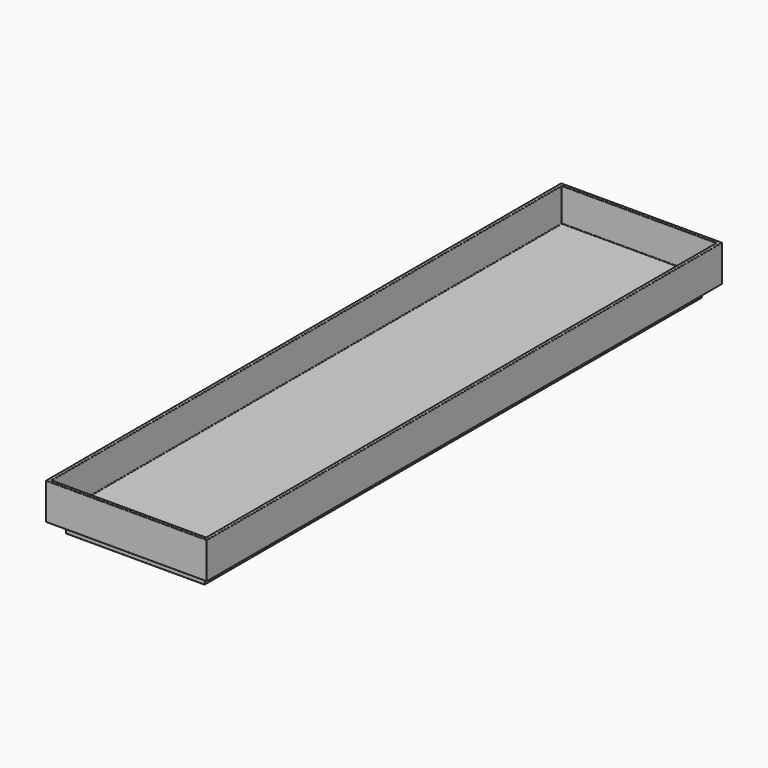
from build123d import *

# Parameters (mm, degrees)
F0_W     = 145
F0_H     = 580
F1_DEPTH = 3
F2_W     = 145
F2_H     = 580
F2_W_2   = 138.9999985695
F2_H_2   = 573.9999985695
F3_DEPTH = 30
F4_W     = 125
F4_H     = 560
F4_W_2   = 119.0000200272
F4_H_2   = 554.0000200272
F5_DEPTH = 10
F6_R     = 0.5


with BuildPart() as f1:
    # F0 (on Top) → F1 (new body)
    with BuildSketch(Plane.XY):
        Rectangle(F0_W, F0_H)
    extrude(amount=F1_DEPTH)

    # F2 (on face) → F3 (join)
    with BuildSketch(Plane.XY.offset(3)):
        Rectangle(F2_W, F2_H)
        Rectangle(F2_W_2, F2_H_2, mode=Mode.SUBTRACT)
    extrude(amount=F3_DEPTH)

    # F4 (on face) → F5 (join)
    with BuildSketch(Plane(origin=(0, 0, 0), x_dir=(1, 0, 0), z_dir=(0, 0, -1))):
        Rectangle(F4_W, F4_H)
        Rectangle(F4_W_2, F4_H_2, mode=Mode.SUBTRACT)
    extrude(amount=F5_DEPTH)

    # F6
    f6_edges = [f1.edges().sort_by_distance(p)[0] for p in [
        (0, 290, 0),
        (72.5, 0, 0),
        (-72.5, 0, 0),
        (0, -290, 0),
        (62.5, 0, 0),
        (0, 280, 0),
        (-62.5, 0, 0),
        (0, -280, 0),
        (59.50001, 0, 0),
        (0, -277.00001, 0),
        (-59.50001, 0, 0),
        (0, 277.00001, 0),
        (-62.5, 280, -5),
        (0, -280, -10),
        (-62.5, 0, -10),
        (0, 280, -10),
        (62.5, 0, -10),
        (0, 277.00001, -10),
        (-59.50001, 0, -10),
        (0, -277.00001, -10),
        (59.50001, 0, -10),
        (59.50001, 277.00001, -5),
        (-59.50001, 277.00001, -5),
        (62.5, -280, -5),
        (-62.5, -280, -5),
        (62.5, 280, -5),
        (-72.5, -290, 16.5),
        (0, -290, 33),
        (72.5, -290, 16.5),
        (72.5, 0, 33),
        (72.5, 290, 16.5),
        (0, 290, 33),
        (-72.5, 290, 16.5),
        (69.499999, 0, 33),
        (0, 286.999999, 3),
        (-69.499999, -286.999999, 18),
        (-69.499999, 286.999999, 18),
        (-69.499999, 0, 3),
        (-69.499999, 0, 33),
        (69.499999, -286.999999, 18),
        (0, -286.999999, 3),
        (0, -286.999999, 33),
        (-72.5, 0, 33),
        (0, 286.999999, 33),
    ]]
    fillet(f6_edges, radius=F6_R)


solid = f1.part
